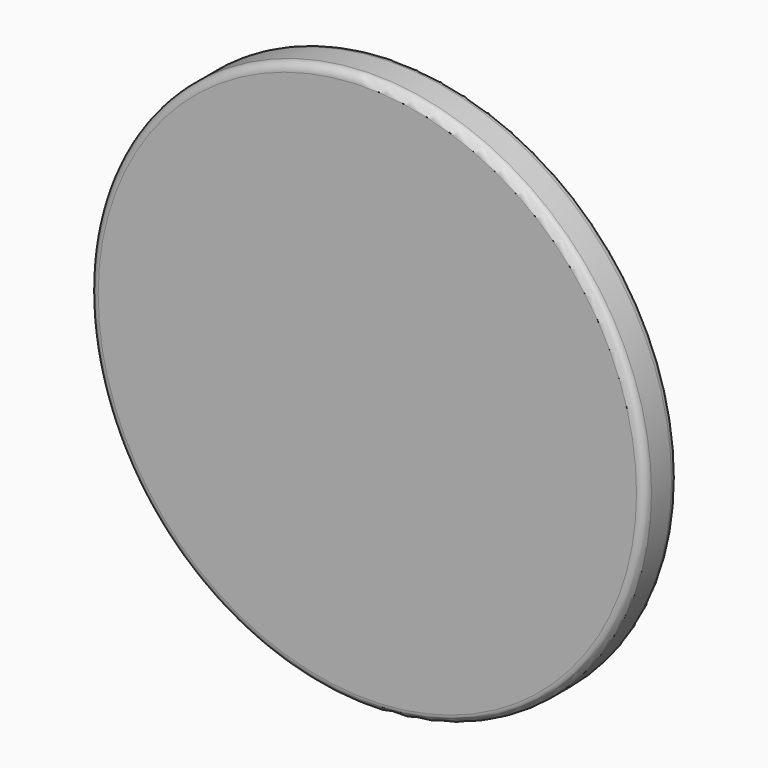
from build123d import *

# Parameters (mm, degrees)
F0_R     = 127
F1_DEPTH = 19.05
F2_R     = 3.81
F3_T     = -2.54


# Not quite as in the source:
# - a shell that OpenCascade refuses in one call is made with other operations: the cavity is built on its own and cut out


with BuildPart() as f1:
    # F0 (on Front) → F1 (new body)
    with BuildSketch(Plane.XZ):
        Circle(F0_R)
    extrude(amount=F1_DEPTH)

    # F2
    f2_edges = [f1.edges().sort_by_distance(p)[0] for p in [
        (-127, 0, 0),
        (-127, -19.05, 0),
    ]]
    fillet(f2_edges, radius=F2_R)

    # F3: a shell. OpenCascade refuses it in one call, so the cavity is built on its own and cut out:
    # the body offset inwards by the wall thickness, plus a prism from it out through each open face.
    f3_core = offset(f1.part, amount=F3_T, mode=Mode.PRIVATE)
    f3_exits = [f3_core.faces().sort_by_distance(p)[0] for p in [
        (0, -2.54, 0),
    ]]
    add(f3_core, mode=Mode.SUBTRACT)
    extrude(f3_exits, amount=-F3_T, mode=Mode.SUBTRACT)


solid = f1.part
